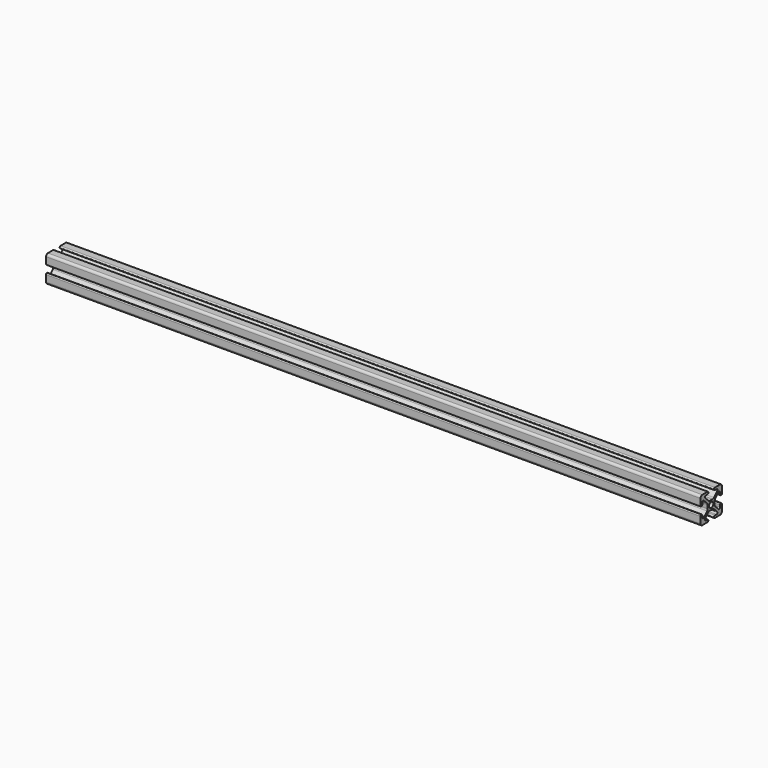
from build123d import *

# Parameters (mm, degrees)
F0_R     = 2.5
F2_DEPTH = 609.6
F3_R     = 2.14
F4_R     = 1.06999


# Not quite as in the source:
# - a fillet or chamfer is up to 0.001 mm smaller than in the source, because OpenCascade refuses the exact size


with BuildPart() as f2:
    # F0 (on Right) → F2 (new body)
    with BuildSketch(Plane.YZ):
        Polygon((2.5367914883, -4.05), (4.05, -4.05), (4.05, -2.5367914883), (4.05, 2.5367914883), (4.05, 4.05), (2.5367914883, 4.05), (-2.5367914883, 4.05), (-4.05, 4.05), (-4.05, 2.5367914883), (-4.05, -2.5367914883), (-4.05, -4.05), (-2.5367914883, -4.05), align=None)
        Circle(F0_R, mode=Mode.SUBTRACT)
        Polygon((-10.36, 8.8467914883), (-4.05, 2.5367914883), (-4.05, 4.05), (-2.5367914883, 4.05), (-8.8467914883, 10.36), (-3.25, 10.36), (-3.25, 12.5), (-12.5, 12.5), (-12.5, 3.25), (-10.36, 3.25), align=None)
        Polygon((4.05, 4.05), (4.05, 2.5367914883), (10.36, 8.8467914883), (10.36, 3.25), (12.5, 3.25), (12.5, 12.5), (3.25, 12.5), (3.25, 10.36), (8.8467914883, 10.36), (2.5367914883, 4.05), align=None)
        Polygon((-8.8467914883, -10.36), (-2.5367914883, -4.05), (-4.05, -4.05), (-4.05, -2.5367914883), (-10.36, -8.8467914883), (-10.36, -3.25), (-12.5, -3.25), (-12.5, -12.5), (-3.25, -12.5), (-3.25, -10.36), align=None)
        Polygon((4.05, -2.5367914883), (4.05, -4.05), (2.5367914883, -4.05), (8.8467914883, -10.36), (3.25, -10.36), (3.25, -12.5), (12.5, -12.5), (12.5, -3.25), (10.36, -3.25), (10.36, -8.8467914883), align=None)
    extrude(amount=F2_DEPTH)

    # F3
    f3_edges = [f2.edges().sort_by_distance(p)[0] for p in [
        (304.8, -12.5, 12.5),
        (304.8, 12.5, 12.5),
        (304.8, 12.5, -12.5),
        (304.8, -12.5, -12.5),
        (304.8, -4.05, 2.536791),
        (304.8, -4.05, -2.536791),
        (304.8, -2.536791, 4.05),
        (304.8, 2.536791, 4.05),
        (304.8, 4.05, 2.536791),
        (304.8, 4.05, -2.536791),
        (304.8, -2.536791, -4.05),
        (304.8, 2.536791, -4.05),
    ]]
    fillet(f3_edges, radius=F3_R)

    # F4 (radius 1.07 in the source; OpenCascade refuses exactly that, so slightly less here)
    f4_edges = [f2.edges().sort_by_distance(p)[0] for p in [
        (304.8, -12.5, 3.25),
        (304.8, -10.36, 3.25),
        (304.8, -3.25, 12.5),
        (304.8, -3.25, 10.36),
        (304.8, 3.25, 12.5),
        (304.8, 3.25, 10.36),
        (304.8, 10.36, 3.25),
        (304.8, 12.5, 3.25),
        (304.8, 10.36, -3.25),
        (304.8, 12.5, -3.25),
        (304.8, 3.25, -10.36),
        (304.8, 3.25, -12.5),
        (304.8, -3.25, -10.36),
        (304.8, -3.25, -12.5),
        (304.8, -10.36, 8.846791),
        (304.8, -8.846791, 10.36),
        (304.8, 8.846791, 10.36),
        (304.8, 10.36, 8.846791),
        (304.8, 8.846791, -10.36),
        (304.8, 10.36, -8.846791),
        (304.8, -8.846791, -10.36),
        (304.8, -10.36, -8.846791),
        (304.8, -10.36, -3.25),
        (304.8, -12.5, -3.25),
    ]]
    fillet(f4_edges, radius=F4_R)


solid = f2.part
